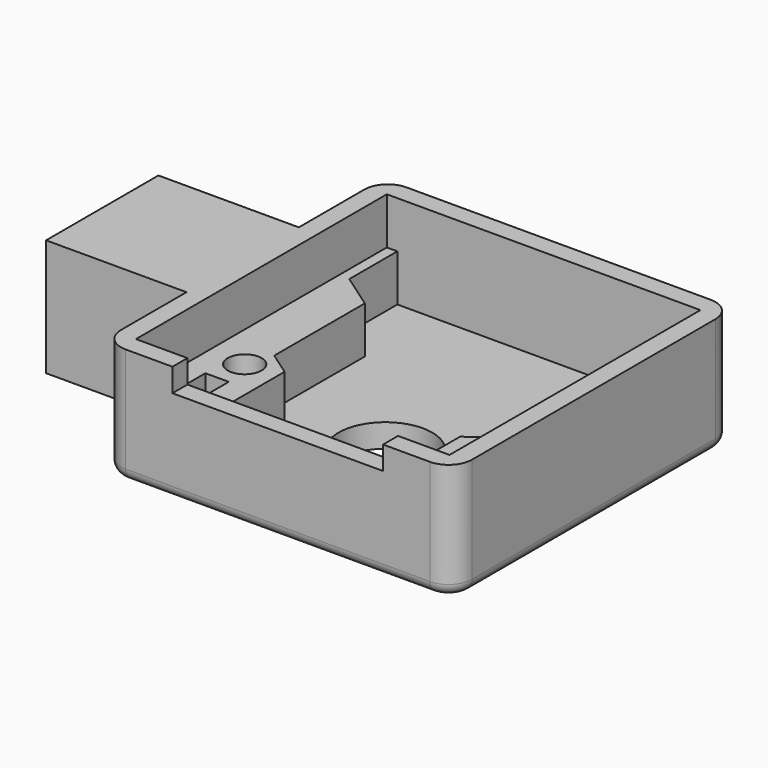
from build123d import *

# Parameters (mm, degrees)
F0_W     = 12
F0_H     = 12
F1_DEPTH = 10
F0_W_2   = 2
F0_H_2   = 3.1217085198
F0_R     = 1.4457822704
F2_DEPTH = 6
F0_R_2   = 4
F0_W_3   = 25
F0_H_3   = 0.9
F3_DEPTH = 2
F5_DEPTH = 12
F6_R     = 2
F7_R     = 1
F8_W     = 18
F8_H     = 1.9928832203
F9_DEPTH = 25


# Not quite as in the source:
# - a feature names something its author has since deleted; it is built from what else it names


with BuildPart() as f1:
    # F0 (on Top) → F1 (new body)
    with BuildSketch(Plane.XY):
        Polygon((15, -15), (15, 15), (-15, 15), (-15, 6), (-15, -6), (-15, -15), align=None)
        Polygon((12.5, 13.4), (13.4, 13.4), (13.4, -13.4), (-13.4, -13.4), (-13.4, 13.4), (-12.5, 13.4), align=None, mode=Mode.SUBTRACT)
        with Locations((-21, 0)):
            Rectangle(F0_W, F0_H)
    extrude(amount=F1_DEPTH)

    # F0 (on Top) → F2 (join)
    with BuildSketch(Plane.XY):
        Polygon((-9.5, -3.5004718229), (-12.5, -1.4055506326), (-12.5, -12.5), (-7.5, -12.5), (-7.5, -4.8970859498), align=None)
        with Locations((-10.5, -9.9175968207)):
            Rectangle(F0_W_2, F0_H_2, mode=Mode.SUBTRACT)
        with Locations((-10.256325826, -5.7152966037)):
            Circle(F0_R, mode=Mode.SUBTRACT)
        Polygon((-9.5, 6.1722276732), (-12.5, 8.2671488635), (-12.5, -1.4055506326), (-9.5, -3.5004718229), align=None)
        Polygon((12.5, -1.4055506326), (12.5, 8.2671488635), (9.5, 6.1722276732), (9.5, -3.5004718229), align=None)
        Polygon((12.5, -12.5), (12.5, -1.4055506326), (9.5, -3.5004718229), (7.5, -4.8970859498), (7.5, -12.5), align=None)
        with Locations((10.5, -9.9175968207)):
            Rectangle(F0_W_2, F0_H_2, mode=Mode.SUBTRACT)
        with Locations((10.256325826, -5.7152966037)):
            Circle(F0_R, mode=Mode.SUBTRACT)
        Polygon((13.4, -13.4), (13.4, 13.4), (12.5, 13.4), (12.5, 12.5), (12.5, 8.2671488635), (12.5, -1.4055506326), (12.5, -12.5), (7.5, -12.5), (-7.5, -12.5), (-12.5, -12.5), (-12.5, -1.4055506326), (-12.5, 8.2671488635), (-12.5, 12.5), (-12.5, 13.4), (-13.4, 13.4), (-13.4, -13.4), align=None)
    extrude(amount=F2_DEPTH)

    # F0 (on Top) → F3 (join)
    with BuildSketch(Plane.XY):
        Polygon((12.5, 8.2671488635), (12.5, 12.5), (-12.5, 12.5), (-12.5, 8.2671488635), (-9.5, 6.1722276732), (-9.5, -3.5004718229), (-7.5, -4.8970859498), (-7.5, -12.5), (7.5, -12.5), (7.5, -4.8970859498), (9.5, -3.5004718229), (9.5, 6.1722276732), align=None)
        with Locations((0, -3.5)):
            Circle(F0_R_2, mode=Mode.SUBTRACT)
        with Locations((10.256325826, -5.7152966037)):
            Circle(F0_R)
        with Locations((10.5, -9.9175968207)):
            Rectangle(F0_W_2, F0_H_2)
        with Locations((-10.5, -9.9175968207)):
            Rectangle(F0_W_2, F0_H_2)
        with Locations((-10.256325826, -5.7152966037)):
            Circle(F0_R)
        with Locations((0, 12.95)):
            Rectangle(F0_W_3, F0_H_3)
    extrude(amount=F3_DEPTH)

    # F4 (on face) → F5 (cut)
    with BuildSketch(Plane(origin=(-27, 0, 0), x_dir=(0, -1, 0), z_dir=(-1, 0, 0))):
        Polygon((-3.6, 5.1207184246), (3.6, 5.1207184246), (0, 8.8730510324), align=None)
        Polygon((0, 1.3683858167), (3.6, 5.1207184246), (-3.6, 5.1207184246), align=None)
    extrude(amount=-F5_DEPTH, mode=Mode.SUBTRACT)

    # F6
    f6_edges = [f1.edges().sort_by_distance(p)[0] for p in [
        (15, 15, 5),
        (-15, 15, 5),
        (-15, -15, 5),
        (15, -15, 5),
    ]]
    fillet(f6_edges, radius=F6_R)

    # F7
    f7_edges = [f1.edges().sort_by_distance(p)[0] for p in [
        (-15, -9.5, 0),
        (0, -15, 0),
    ]]
    fillet(f7_edges, radius=F7_R)

    # F8 (on face) → F9 (cut)
    with BuildSketch(Plane.XZ.offset(15)):
        with Locations((0, 9.0035583898)):
            Rectangle(F8_W, F8_H)
    extrude(amount=-F9_DEPTH, mode=Mode.SUBTRACT)


solid = f1.part
